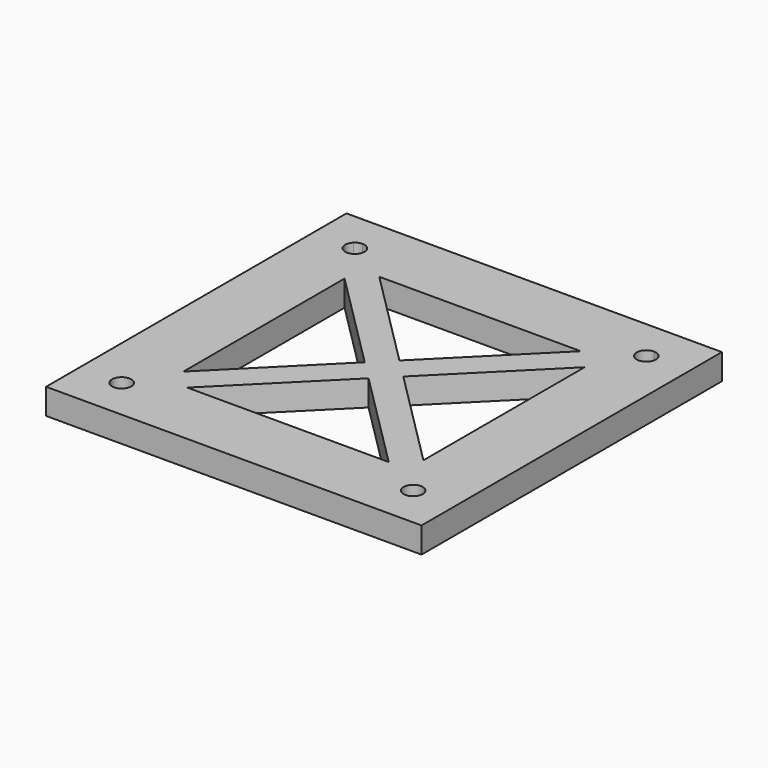
from build123d import *
from build123d import SkipClean  # not in build123d's __all__

# Parameters (mm, degrees)
F1_DEPTH = 4
F2_DEPTH = 2


with BuildPart() as f1:
    # F0 (on Top) → F1 (new body)
    with BuildSketch(Plane.XY):
        Polygon((0, -51.35), (-3.5355339059, -54.8855339059), (54.8855339059, -54.8855339059), (51.35, -51.35), (48.35, -51.35), (44.35, -51.35), (7, -51.35), (3, -51.35), align=None)
        Polygon((7, -7), (0, -7), (0, -44.35), (7, -44.35), (7, -41.3499993608), (7, -10), align=None)
        Polygon((10.0000006392, -44.35), (7, -44.35), (7, -51.35), (44.35, -51.35), (44.35, -44.35), (41.35, -44.35), align=None)
        with BuildLine():
            Line((7, -44.35), (0, -44.35))
            Line((0, -44.35), (0, -48.35))
            Line((0, -48.35), (1.5, -48.35))
            ThreePointArc((1.5, -48.35), (3, -46.85), (4.5, -48.35))
            ThreePointArc((4.5, -48.35), (4.0606601718, -49.4106601718), (3, -49.85))
            Line((3, -49.85), (3, -51.35))
            Line((3, -51.35), (7, -51.35))
            Line((7, -51.35), (7, -44.35))
        make_face()
        with BuildLine():
            Line((0, -48.35), (0, -51.35))
            Line((0, -51.35), (3, -51.35))
            Line((3, -51.35), (3, -49.85))
            ThreePointArc((3, -49.85), (1.9393398282, -49.4106601718), (1.5, -48.35))
            Line((1.5, -48.35), (0, -48.35))
        make_face()
        Polygon((0, -3), (0, 0), (-3.5355339059, 3.5355339059), (-3.5355339059, -54.8855339059), (0, -51.35), (0, -48.35), (0, -44.35), (0, -7), align=None)
        with BuildLine():
            Line((7, 0), (3, 0))
            Line((3, 0), (3, -1.5))
            ThreePointArc((3, -1.5), (4.0606601718, -1.9393398282), (4.5, -3))
            ThreePointArc((4.5, -3), (3, -4.5), (1.5, -3))
            Line((1.5, -3), (0, -3))
            Line((0, -3), (0, -7))
            Line((0, -7), (7, -7))
            Line((7, -7), (7, 0))
        make_face()
        with BuildLine():
            Line((3, 0), (0, 0))
            Line((0, 0), (1.9393398282, -1.9393398282))
            ThreePointArc((1.9393398282, -1.9393398282), (2.4259748515, -1.6141807012), (3, -1.5))
            Line((3, -1.5), (3, 0))
        make_face()
        with BuildLine():
            Line((1.9393398282, -1.9393398282), (0, 0))
            Line((0, 0), (0, -3))
            Line((0, -3), (1.5, -3))
            ThreePointArc((1.5, -3), (1.6141807012, -2.4259748515), (1.9393398282, -1.9393398282))
        make_face()
        Polygon((-3.5355339059, 3.5355339059), (0, 0), (3, 0), (7, 0), (44.35, 0), (48.35, 0), (51.35, 0), (54.8855339059, 3.5355339059), align=None)
        Polygon((44.35, 0), (7, 0), (7, -7), (10, -7), (41.3499993608, -7), (44.35, -7), align=None)
        with BuildLine():
            Line((48.35, 0), (44.35, 0))
            Line((44.35, 0), (44.35, -7))
            Line((44.35, -7), (51.35, -7))
            Line((51.35, -7), (51.35, -3))
            Line((51.35, -3), (49.85, -3))
            ThreePointArc((49.85, -3), (47.2893398282, -4.0606601718), (48.35, -1.5))
            Line((48.35, -1.5), (48.35, 0))
        make_face()
        with BuildLine():
            Line((51.35, -3), (51.35, 0))
            Line((51.35, 0), (48.35, 0))
            Line((48.35, 0), (48.35, -1.5))
            ThreePointArc((48.35, -1.5), (49.4106601718, -1.9393398282), (49.85, -3))
            Line((49.85, -3), (51.35, -3))
        make_face()
        Polygon((54.8855339059, -54.8855339059), (54.8855339059, 3.5355339059), (51.35, 0), (51.35, -3), (51.35, -7), (51.35, -44.35), (51.35, -48.35), (51.35, -51.35), align=None)
        Polygon((51.35, -7), (44.35, -7), (44.35, -10.0000006392), (44.35, -41.35), (44.35, -44.35), (51.35, -44.35), align=None)
        with BuildLine():
            Line((48.35, -51.35), (51.35, -51.35))
            Line((51.35, -51.35), (51.35, -48.35))
            Line((51.35, -48.35), (49.85, -48.35))
            ThreePointArc((49.85, -48.35), (49.4106601718, -49.4106601718), (48.35, -49.85))
            Line((48.35, -49.85), (48.35, -51.35))
        make_face()
        with BuildLine():
            Line((44.35, -51.35), (48.35, -51.35))
            Line((48.35, -51.35), (48.35, -49.85))
            ThreePointArc((48.35, -49.85), (47.2893398282, -47.2893398282), (49.85, -48.35))
            Line((49.85, -48.35), (51.35, -48.35))
            Line((51.35, -48.35), (51.35, -44.35))
            Line((51.35, -44.35), (44.35, -44.35))
            Line((44.35, -44.35), (44.35, -51.35))
        make_face()
        Polygon((7, -41.3499993608), (7, -44.35), (8.5000003196, -42.8499996804), align=None)
        Polygon((8.5000003196, -42.8499996804), (7, -44.35), (10.0000006392, -44.35), align=None)
        Polygon((8.5000003196, -42.8499996804), (10.0000006392, -44.35), (25.6750003196, -28.6750003196), (24.175, -27.175), align=None)
        Polygon((22.6749996804, -25.6749996804), (7, -41.3499993608), (8.5000003196, -42.8499996804), (24.175, -27.175), align=None)
        Polygon((8.5, -8.5), (7, -10), (22.6749996804, -25.6749996804), (24.1749996804, -24.1749996804), align=None)
        Polygon((25.6749996804, -22.6749996804), (10, -7), (8.5, -8.5), (24.1749996804, -24.1749996804), align=None)
        Polygon((27.175, -24.175), (25.6749996804, -22.6749996804), (24.1749996804, -24.1749996804), (25.675, -25.675), align=None)
        Polygon((27.1750003196, -27.1750003196), (28.6750003196, -25.6750003196), (27.175, -24.175), (25.675, -25.675), align=None)
        Polygon((25.675, -25.675), (24.175, -27.175), (25.6750003196, -28.6750003196), (27.1750003196, -27.1750003196), align=None)
        Polygon((24.1749996804, -24.1749996804), (22.6749996804, -25.6749996804), (24.175, -27.175), (25.675, -25.675), align=None)
        Polygon((25.6750003196, -28.6750003196), (41.35, -44.35), (42.85, -42.85), (27.1750003196, -27.1750003196), align=None)
        Polygon((42.85, -42.85), (44.35, -41.35), (28.6750003196, -25.6750003196), (27.1750003196, -27.1750003196), align=None)
        Polygon((8.5, -8.5), (7, -7), (7, -10), align=None)
        Polygon((10, -7), (7, -7), (8.5, -8.5), align=None)
        Polygon((28.6750003196, -25.6750003196), (44.35, -10.0000006392), (42.8499996804, -8.5000003196), (27.175, -24.175), align=None)
        Polygon((42.8499996804, -8.5000003196), (41.3499993608, -7), (25.6749996804, -22.6749996804), (27.175, -24.175), align=None)
        Polygon((44.35, -10.0000006392), (44.35, -7), (42.8499996804, -8.5000003196), align=None)
        Polygon((44.35, -44.35), (44.35, -41.35), (42.85, -42.85), align=None)
        Polygon((42.85, -42.85), (41.35, -44.35), (44.35, -44.35), align=None)
        Polygon((42.8499996804, -8.5000003196), (44.35, -7), (41.3499993608, -7), align=None)
    extrude(amount=F1_DEPTH)

    # F0 (on Top) → F2 (join)
    with BuildSketch(Plane.XY):
        with BuildLine():
            Line((7, -44.35), (0, -44.35))
            Line((0, -44.35), (0, -48.35))
            Line((0, -48.35), (1.5, -48.35))
            ThreePointArc((1.5, -48.35), (3, -46.85), (4.5, -48.35))
            ThreePointArc((4.5, -48.35), (4.0606601718, -49.4106601718), (3, -49.85))
            Line((3, -49.85), (3, -51.35))
            Line((3, -51.35), (7, -51.35))
            Line((7, -51.35), (7, -44.35))
        make_face()
        with BuildLine():
            Line((0, -48.35), (0, -51.35))
            Line((0, -51.35), (3, -51.35))
            Line((3, -51.35), (3, -49.85))
            ThreePointArc((3, -49.85), (1.9393398282, -49.4106601718), (1.5, -48.35))
            Line((1.5, -48.35), (0, -48.35))
        make_face()
        with BuildLine():
            Line((44.35, -51.35), (48.35, -51.35))
            Line((48.35, -51.35), (48.35, -49.85))
            ThreePointArc((48.35, -49.85), (47.2893398282, -47.2893398282), (49.85, -48.35))
            Line((49.85, -48.35), (51.35, -48.35))
            Line((51.35, -48.35), (51.35, -44.35))
            Line((51.35, -44.35), (44.35, -44.35))
            Line((44.35, -44.35), (44.35, -51.35))
        make_face()
        with BuildLine():
            Line((48.35, -51.35), (51.35, -51.35))
            Line((51.35, -51.35), (51.35, -48.35))
            Line((51.35, -48.35), (49.85, -48.35))
            ThreePointArc((49.85, -48.35), (49.4106601718, -49.4106601718), (48.35, -49.85))
            Line((48.35, -49.85), (48.35, -51.35))
        make_face()
        with BuildLine():
            Line((48.35, 0), (44.35, 0))
            Line((44.35, 0), (44.35, -7))
            Line((44.35, -7), (51.35, -7))
            Line((51.35, -7), (51.35, -3))
            Line((51.35, -3), (49.85, -3))
            ThreePointArc((49.85, -3), (47.2893398282, -4.0606601718), (48.35, -1.5))
            Line((48.35, -1.5), (48.35, 0))
        make_face()
        with BuildLine():
            Line((51.35, -3), (51.35, 0))
            Line((51.35, 0), (48.35, 0))
            Line((48.35, 0), (48.35, -1.5))
            ThreePointArc((48.35, -1.5), (49.4106601718, -1.9393398282), (49.85, -3))
            Line((49.85, -3), (51.35, -3))
        make_face()
        with BuildLine():
            Line((7, 0), (3, 0))
            Line((3, 0), (3, -1.5))
            ThreePointArc((3, -1.5), (4.0606601718, -1.9393398282), (4.5, -3))
            ThreePointArc((4.5, -3), (3, -4.5), (1.5, -3))
            Line((1.5, -3), (0, -3))
            Line((0, -3), (0, -7))
            Line((0, -7), (7, -7))
            Line((7, -7), (7, 0))
        make_face()
        with BuildLine():
            Line((1.9393398282, -1.9393398282), (0, 0))
            Line((0, 0), (0, -3))
            Line((0, -3), (1.5, -3))
            ThreePointArc((1.5, -3), (1.6141807012, -2.4259748515), (1.9393398282, -1.9393398282))
        make_face()
        with BuildLine():
            Line((3, 0), (0, 0))
            Line((0, 0), (1.9393398282, -1.9393398282))
            ThreePointArc((1.9393398282, -1.9393398282), (2.4259748515, -1.6141807012), (3, -1.5))
            Line((3, -1.5), (3, 0))
        make_face()
    with SkipClean():  # cleaning this boolean's faces spoils the solid; the shape is the same uncleaned
        extrude(amount=-F2_DEPTH)


solid = f1.part
